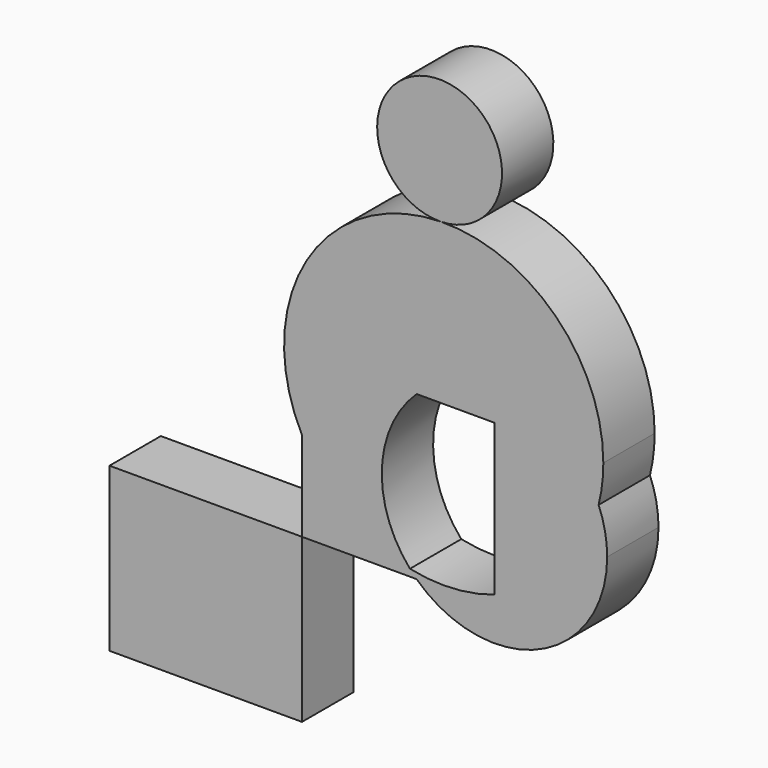
from build123d import *

# Parameters (mm, degrees)
F1_DEPTH = 25
F0_W     = 75
F0_H     = 63.5


with BuildPart() as f1:
    # F0 (on Front) → F1 (new body)
    with BuildSketch(Plane.XZ):
        with BuildLine():
            Line((0, 34.8829194066), (0, 0))
            Line((0, 0), (44.6694262963, 0))
            ThreePointArc((44.6694262963, 0), (43.3351861339, 1.3305035541), (42.0592569414, 2.7170248176))
            ThreePointArc((42.0592569414, 2.7170248176), (17.4353764526, 14.100225033), (0, 34.8829194066))
        make_face()
        with BuildLine():
            ThreePointArc((42.0592569414, 2.7170248176), (43.3351861339, 1.3305035541), (44.6694262963, 0))
            Line((44.6694262963, 0), (75, 0))
            Line((75, 0), (75, 4.5406466367))
            ThreePointArc((75, 4.5406466367), (58.6527595412, 1.4046744939), (42.0592569414, 2.7170248176))
        make_face()
        with BuildLine():
            Line((75, 0), (44.6694262963, 0))
            ThreePointArc((44.6694262963, 0), (92.2658477308, -8.6219791852), (118.9090674143, 31.75))
            ThreePointArc((118.9090674143, 31.75), (118.0679163411, 40.3034076971), (115.5766904116, 48.5291059488))
            ThreePointArc((115.5766904116, 48.5291059488), (100.9273669379, 21.3332201623), (75, 4.5406466367))
            Line((75, 4.5406466367), (75, 0))
        make_face()
        with BuildLine():
            ThreePointArc((54.0630152571, 125.6797351802), (1.7798186625, 95.3169035326), (0, 34.8829194066))
            Line((0, 34.8829194066), (0, 63.5))
            Line((0, 63.5), (44.6694262963, 63.5))
            ThreePointArc((44.6694262963, 63.5), (84.0707025125, 74.7119431256), (115.5766904116, 48.5291059488))
            ThreePointArc((115.5766904116, 48.5291059488), (116.9466255151, 55.9589073111), (117.4055280417, 63.5))
            ThreePointArc((117.4055280417, 63.5), (98.7811445192, 107.8807204565), (54.0630152571, 125.6797351802))
        make_face()
        with BuildLine():
            Line((0, 63.5), (0, 34.8829194066))
            ThreePointArc((0, 34.8829194066), (17.4353764526, 14.100225033), (42.0592569414, 2.7170248176))
            ThreePointArc((42.0592569414, 2.7170248176), (31.1313620086, 33.6338264198), (44.6694262963, 63.5))
            Line((44.6694262963, 63.5), (0, 63.5))
        make_face()
        with BuildLine():
            Line((75, 63.5), (75, 4.5406466367))
            ThreePointArc((75, 4.5406466367), (100.9273669379, 21.3332201623), (115.5766904116, 48.5291059488))
            ThreePointArc((115.5766904116, 48.5291059488), (84.0707025125, 74.7119431256), (44.6694262963, 63.5))
            Line((44.6694262963, 63.5), (75, 63.5))
        make_face()
    extrude(amount=F1_DEPTH)


with BuildPart() as f1b:
    # F0 (on Front) → F1, piece 2 (new body)
    with BuildSketch(Plane.XZ):
        with BuildLine():
            ThreePointArc((77.9391215075, 150.0023305416), (36.2521247684, 167.0438760613), (54.0630152571, 125.6797351802))
            ThreePointArc((54.0630152571, 125.6797351802), (70.9725780667, 132.9607850219), (77.9391215075, 150.0023305416))
        make_face()
    extrude(amount=F1_DEPTH)


with BuildPart() as f1c:
    # F0 (on Front) → F1, piece 3 (new body)
    with BuildSketch(Plane.XZ):
        with Locations((-37.5, -31.75)):
            Rectangle(F0_W, F0_H)
    extrude(amount=F1_DEPTH)


solid = Compound([f1.part, f1b.part, f1c.part])
